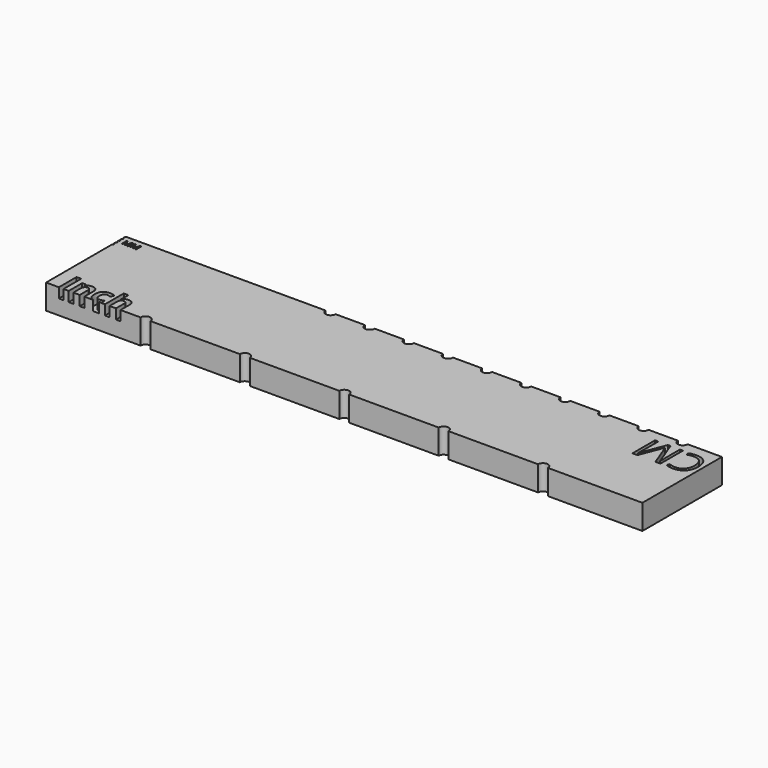
from build123d import *

# Parameters (mm, degrees)
F0_W          = 152.4
F0_H          = 25.4
F1_DEPTH      = 6.35
F2_R          = 1.27
F3_DEPTH      = 25.4
F4_TEXT_SIZE  = 7.9033747574
F5_DEPTH      = 2.54
F6_TEXT_SIZE  = 10.1079372909
F7_DEPTH      = 2.54
F8_R          = 1.27
F9_DEPTH      = 2.54
F10_R         = 0.254
F11_DEPTH     = 2.54
F12_TEXT_SIZE = 2.3443588159
F13_DEPTH     = 2.54


# Not quite as in the source:
# - Text() gives the source's letters only with a copy of the font that has no kerning and outlines rounded to 1/6400 em; it was checked with that copy


with BuildPart() as f1:
    # F0 (on Top) → F1 (new body)
    with BuildSketch(Plane.XY):
        with Locations((76.2, 12.7)):
            Rectangle(F0_W, F0_H)
    extrude(amount=F1_DEPTH)

    # F2 (on face) → F3 (cut)
    with BuildSketch(Plane.XY.offset(6.35)):
        with Locations((25.4, 0)):
            Circle(F2_R)
        with Locations((50.8, 0)):
            Circle(F2_R)
        with Locations((76.2, 0)):
            Circle(F2_R)
        with Locations((101.6, 0)):
            Circle(F2_R)
        with Locations((127, 0)):
            Circle(F2_R)
    extrude(amount=-F3_DEPTH, mode=Mode.SUBTRACT)

    # F4 (on face) → F5 (cut)
    with BuildSketch(Plane.XY.offset(6.35)):
        with Locations((2.5562504306, 0)):
            Text('Inch', F4_TEXT_SIZE, font='Open Sans', font_style=FontStyle.BOLD, text_align=(TextAlign.LEFT, TextAlign.BOTTOM))
    extrude(amount=-F5_DEPTH, mode=Mode.SUBTRACT)

    # F6 (on face) → F7 (cut)
    with BuildSketch(Plane.XY.offset(6.35)):
        with Locations(Location((152.0068049431, 22.6673576981), (0, 0, -180))):
            Text('CM', F6_TEXT_SIZE, font='Open Sans', text_align=(TextAlign.LEFT, TextAlign.BOTTOM))
    extrude(amount=-F7_DEPTH, mode=Mode.SUBTRACT)

    # F8 (on face) → F9 (cut)
    with BuildSketch(Plane.XY.offset(6.35)):
        with Locations((142.4, 25.4)):
            Circle(F8_R)
        with Locations((132.4, 25.4)):
            Circle(F8_R)
        with Locations((122.4, 25.4)):
            Circle(F8_R)
        with Locations((112.4, 25.4)):
            Circle(F8_R)
        with Locations((52.4, 25.4)):
            Circle(F8_R)
        with Locations((102.4, 25.4)):
            Circle(F8_R)
        with Locations((92.4, 25.4)):
            Circle(F8_R)
        with Locations((82.4, 25.4)):
            Circle(F8_R)
        with Locations((72.4, 25.4)):
            Circle(F8_R)
        with Locations((62.4, 25.4)):
            Circle(F8_R)
    extrude(amount=-F9_DEPTH, mode=Mode.SUBTRACT)

    # F10 (on face) → F11 (cut)
    with BuildSketch(Plane.XY.offset(6.35)):
        with Locations((0, 25.4)):
            Circle(F10_R)
        with Locations((0, 24.4)):
            Circle(F10_R)
        with Locations((0, 23.4)):
            Circle(F10_R)
        with Locations((0, 22.4)):
            Circle(F10_R)
        with Locations((0, 21.4)):
            Circle(F10_R)
    extrude(amount=-F11_DEPTH, mode=Mode.SUBTRACT)

    # F12 (on face) → F13 (cut)
    with BuildSketch(Plane.XY.offset(6.35)):
        with Locations((1.0993076721, 22.3960727453)):
            Text('MM', F12_TEXT_SIZE, font='Open Sans', text_align=(TextAlign.LEFT, TextAlign.BOTTOM))
    extrude(amount=-F13_DEPTH, mode=Mode.SUBTRACT)


solid = f1.part
